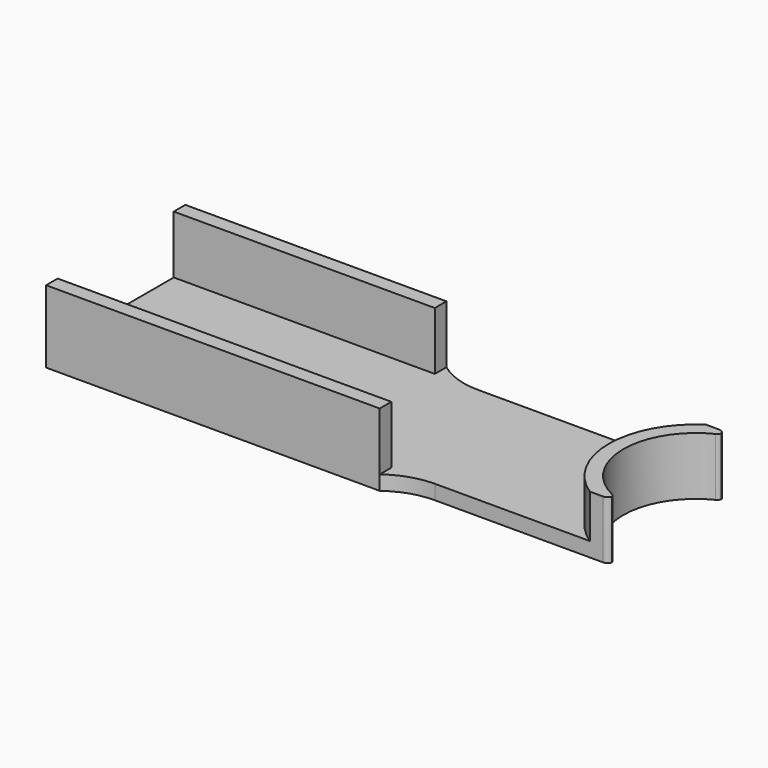
from build123d import *

# Parameters (mm, degrees)
F1_DEPTH    = 5
F3_DEPTH    = 4
F4_W        = 15
F4_H        = 1
F4_W_2      = 20
F5_DEPTH    = 25
F6_T1_DEPTH = 6.2738947701
F6_T3_DEPTH = 7
F8_DEPTH    = 1
F9_T1_DEPTH = 1


# Not quite as in the source:
# - a fillet or chamfer that OpenCascade refuses, or shapes differently, is made with other operations: its cross-section is extruded or revolved along the edge and cut away or added


with BuildPart() as f1:
    # F0 (on Top) → F1 (new body)
    with BuildSketch(Plane.XY):
        with BuildLine():
            Line((38, 0), (0, 0))
            Line((0, 0), (0, -12))
            Line((0, -12), (38, -12))
            Line((38, -12), (38, -10.582575695))
            ThreePointArc((38, -10.582575695), (35, -6), (38, -1.417424305))
            Line((38, -1.417424305), (38, 0))
        make_face()
    extrude(amount=F1_DEPTH)

    # F2 (on face) → F3 (cut)
    with BuildSketch(Plane.XY.offset(5)):
        with BuildLine():
            ThreePointArc((38, -11.6568542495), (34, -6), (38, -0.3431457505))
            Line((38, -0.3431457505), (38, 0))
            Line((38, 0), (18, 0))
            Line((18, 0), (18, -1))
            Line((18, -1), (0, -1))
            Line((0, -1), (0, -11))
            Line((0, -11), (23, -11))
            Line((23, -11), (23, -12))
            Line((23, -12), (38, -12))
            Line((38, -12), (38, -11.6568542495))
        make_face()
    extrude(amount=-F3_DEPTH, mode=Mode.SUBTRACT)

    # F4 (on face) → F5 (cut)
    with BuildSketch(Plane(origin=(0, 0, 0), x_dir=(1, 0, 0), z_dir=(0, 0, -1))):
        with Locations((30.5, 11.5)):
            Rectangle(F4_W, F4_H)
        with Locations((28, 0.5)):
            Rectangle(F4_W_2, F4_H)
    extrude(amount=-F5_DEPTH, mode=Mode.SUBTRACT)

    # F6: fillet of radius 0.4 on 4 edges, made by hand

    # F6_s2 → F6_t1 (cut)
    with BuildSketch(Plane.XY.offset(-0.6369473851)):
        with BuildLine():
            ThreePointArc((37.7777777778, -10.4790320824), (37.9399346342, -10.6265361383), (38, -10.837354649))
            Line((38, -10.837354649), (38, -10.582575695))
            ThreePointArc((38, -10.582575695), (37.8882541717, -10.5321660998), (37.7777777778, -10.4790320824))
        make_face()
        with BuildLine():
            ThreePointArc((38, -1.162645351), (37.9399346342, -1.3734638617), (37.7777777778, -1.5209679176))
            ThreePointArc((37.7777777778, -1.5209679176), (37.8882541717, -1.4678339002), (38, -1.417424305))
            Line((38, -1.417424305), (38, -1.162645351))
        make_face()
    extrude(amount=F6_T1_DEPTH, mode=Mode.SUBTRACT)

    # F6_s4 → F6_t3 (cut)
    with BuildSketch(Plane.XY.offset(-1)):
        with BuildLine():
            ThreePointArc((38, -10.6), (37.8828427125, -10.8828427125), (37.6, -11))
            Line((37.6, -11), (38, -11))
            Line((38, -11), (38, -10.6))
        make_face()
        with BuildLine():
            ThreePointArc((38, -1.4), (37.8828427125, -1.1171572875), (37.6, -1))
            Line((37.6, -1), (38, -1))
            Line((38, -1), (38, -1.4))
        make_face()
    extrude(amount=F6_T3_DEPTH, mode=Mode.SUBTRACT)

    # F7 (on face) → F8 (cut)
    with BuildSketch(Plane.XY.offset(5)):
        with BuildLine():
            ThreePointArc((36.6833752096, -1), (34, -6), (36.6833752096, -11))
            Line((36.6833752096, -11), (37.6, -11))
            ThreePointArc((37.6, -11), (37.8372014652, -10.9220799045), (37.9819891264, -10.7186773245))
            ThreePointArc((37.9819891264, -10.7186773245), (37.9044539493, -10.5779171946), (37.7777777778, -10.4790320824))
            ThreePointArc((37.7777777778, -10.4790320824), (35, -6), (37.7777777778, -1.5209679176))
            ThreePointArc((37.7777777778, -1.5209679176), (37.9044539493, -1.4220828054), (37.9819891264, -1.2813226755))
            ThreePointArc((37.9819891264, -1.2813226755), (37.8372014652, -1.0779200955), (37.6, -1))
            Line((37.6, -1), (36.6833752096, -1))
        make_face()
    extrude(amount=-F8_DEPTH, mode=Mode.SUBTRACT)

    # F9: fillet of radius 5 on 2 edges, made by hand

    # F9_s2 → F9_t1 (join)
    with BuildSketch(Plane.XY):
        with BuildLine():
            ThreePointArc((18, 0), (19.4188611699, -0.7434164903), (21, -1))
            Line((21, -1), (18, -1))
            Line((18, -1), (18, 0))
        make_face()
        with BuildLine():
            ThreePointArc((26, -11), (24.4188611699, -11.2565835097), (23, -12))
            Line((23, -12), (23, -11))
            Line((23, -11), (26, -11))
        make_face()
    extrude(amount=F9_T1_DEPTH)


solid = f1.part
